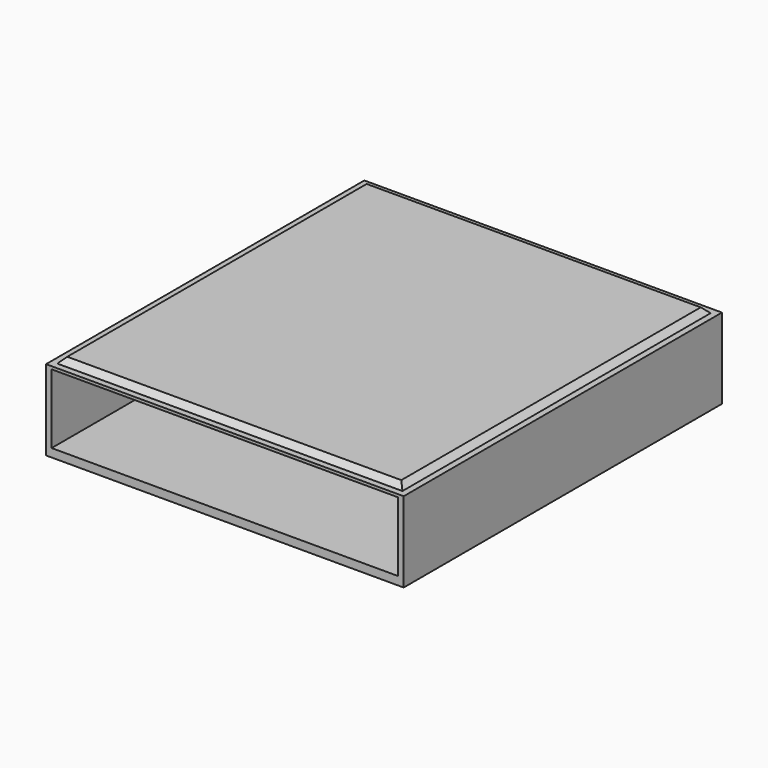
from build123d import *

# Parameters (mm, degrees)
F0_W      = 129
F0_H      = 143.5
F0_W_2    = 125
F0_H_2    = 139.5
F1_DEPTH  = 3
F2_DEPTH  = 2
F3_SIZE   = 1.99999
F5_DEPTH  = 25
F6_W      = 125
F6_H      = 141.5
F6_W_2    = 124.5
F6_H_2    = 139
F6_W_3    = 122.5
F6_H_3    = 137
F7_DEPTH  = 1
F8_DEPTH  = 3
F9_SIZE   = 1.99999
F10_DEPTH = 2
F10_TAPER = 45


# Not quite as in the source:
# - a fillet or chamfer is up to 0.001 mm smaller than in the source, because OpenCascade refuses the exact size
# - a feature names something its author has since deleted; it is built from what else it names


with BuildPart() as f1:
    # F0 (on Top) → F1 (new body)
    with BuildSketch(Plane.XY):
        Rectangle(F0_W, F0_H)
        Rectangle(F0_W_2, F0_H_2, mode=Mode.SUBTRACT)
        Rectangle(F0_W_2, F0_H_2)
    extrude(amount=F1_DEPTH)

    # F0 (on Top) → F2 (cut)
    with BuildSketch(Plane.XY):
        Rectangle(F0_W_2, F0_H_2)
    extrude(amount=F2_DEPTH, mode=Mode.SUBTRACT)

    # F3 (size 2 in the source; OpenCascade refuses exactly that, so slightly less here)
    f3_edges = [f1.edges().sort_by_distance(p)[0] for p in [
        (0, -69.75, 2),
        (62.5, 0, 2),
        (0, 69.75, 2),
        (-62.5, 0, 2),
    ]]
    chamfer(f3_edges, length=F3_SIZE)

    # F4 (on face) → F5 (join)
    with BuildSketch(Plane.XY.offset(3)):
        Polygon((-64.5, 71.75), (-64.5, -71.75), (-62.5, -71.75), (-62.5, 69.75), (62.5, 69.75), (62.5, -71.75), (64.5, -71.75), (64.5, 71.75), align=None)
    extrude(amount=F5_DEPTH)

    # F6 (on face) → F7 (join)
    with BuildSketch(Plane.XY.offset(28)):
        with Locations((0, -1)):
            Rectangle(F6_W, F6_H)
        Rectangle(F6_W_2, F6_H_2, mode=Mode.SUBTRACT)
        Rectangle(F6_W_2, F6_H_2)
        Rectangle(F6_W_3, F6_H_3, mode=Mode.SUBTRACT)
        Rectangle(F6_W_3, F6_H_3)
        Polygon((-64.5, 71.75), (-64.5, -71.75), (-62.5, -71.75), (-62.5, 69.75), (62.5, 69.75), (62.5, -71.75), (64.5, -71.75), (64.5, 71.75), align=None)
    extrude(amount=F7_DEPTH)

    # F6 (on face) → F8 (join)
    with BuildSketch(Plane.XY.offset(28)):
        Rectangle(F6_W_2, F6_H_2)
        Rectangle(F6_W_3, F6_H_3, mode=Mode.SUBTRACT)
        Rectangle(F6_W_3, F6_H_3)
    extrude(amount=F8_DEPTH)

    # F9 (size 2 in the source; OpenCascade refuses exactly that, so slightly less here)
    f9_edges = [f1.edges().sort_by_distance(p)[0] for p in [
        (-62.25, 0, 31),
        (0, 69.5, 31),
        (0, -69.5, 31),
        (62.25, 0, 31),
    ]]
    chamfer(f9_edges, length=F9_SIZE)

    # F6 (on face) → F10 (cut)
    with BuildSketch(Plane.XY.offset(28)):
        Rectangle(F6_W_3, F6_H_3)
    extrude(amount=F10_DEPTH, taper=F10_TAPER, mode=Mode.SUBTRACT)


solid = f1.part
